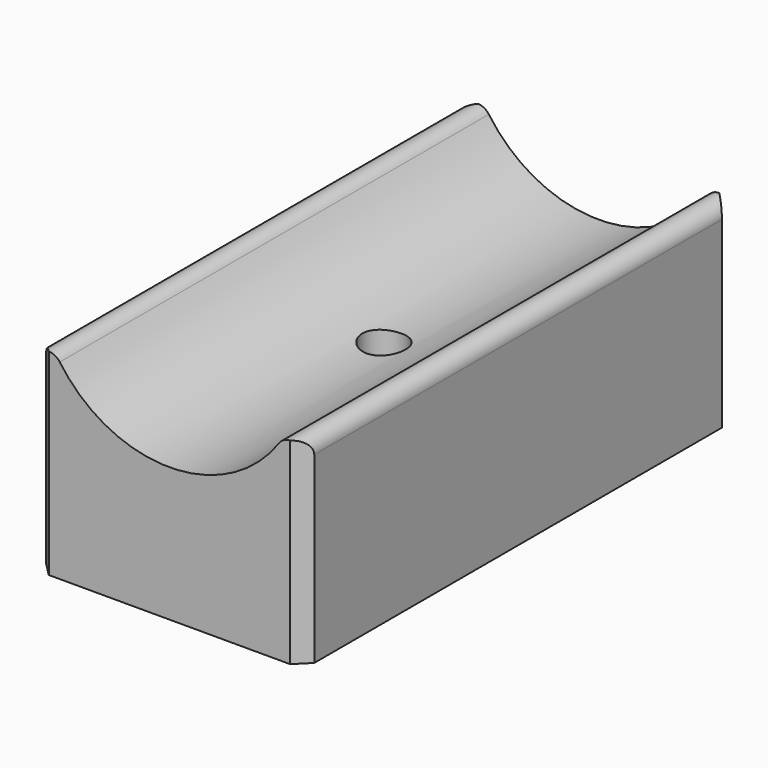
from build123d import *

# Parameters (mm, degrees)
F0_W        = 25.4
F0_H        = 50.8
F1_DEPTH    = 25.4
F3_DEPTH    = 50.8
F5_D        = 4.1
F6_F1_R     = 1.27
F6_F2_R     = 1.27
F7_T1_DEPTH = 23.8998895326


# Not quite as in the source:
# - a fillet or chamfer that OpenCascade refuses, or shapes differently, is made with other operations: its cross-section is extruded or revolved along the edge and cut away or added


with BuildPart() as f1:
    # F0 (on Top) → F1 (new body)
    with BuildSketch(Plane.XY):
        with Locations((12.7, -25.4)):
            Rectangle(F0_W, F0_H)
    extrude(amount=F1_DEPTH)

    # F2 (on face) → F3 (cut)
    with BuildSketch(Plane.XZ.offset(50.8)):
        with BuildLine():
            ThreePointArc((0, 25.4), (12.7, 12.7), (25.4, 25.4))
            Line((25.4, 25.4), (0, 25.4))
        make_face()
    extrude(amount=-F3_DEPTH, mode=Mode.SUBTRACT)

    # F5 (through all)
    with Locations(Plane(origin=(0, 0, 0), x_dir=(1, 0, 0), z_dir=(0, 0, -1))):
        with Locations((12.7, 25.4)):
            Hole(F5_D / 2)

    # F6: fillet of radius 1.27 on 2 edges, made by hand

    # F6_f1
    f6_f1_edges = [f1.edges().sort_by_distance(p)[0] for p in [
        (0, -25.4, 25.4),
    ]]
    fillet(f6_f1_edges, radius=F6_F1_R)

    # F6_f2
    f6_f2_edges = [f1.edges().sort_by_distance(p)[0] for p in [
        (25.4, -25.4, 25.4),
    ]]
    fillet(f6_f2_edges, radius=F6_F2_R)

    # F7: chamfer of 1.27 on 4 edges, made by hand

    # F7_s2 → F7_t1 (cut)
    with BuildSketch(Plane.XY.offset(-3.2660373947)):
        Polygon((25.4, -49.53), (24.13, -50.8), (25.4, -50.8), align=None)
        Polygon((0, -49.53), (1.27, -50.8), (0, -50.8), align=None)
        Polygon((24.13, 0), (25.4, -1.27), (25.4, 0), align=None)
        Polygon((1.27, 0), (0, -1.27), (0, 0), align=None)
    extrude(amount=F7_T1_DEPTH, mode=Mode.SUBTRACT)


solid = f1.part
